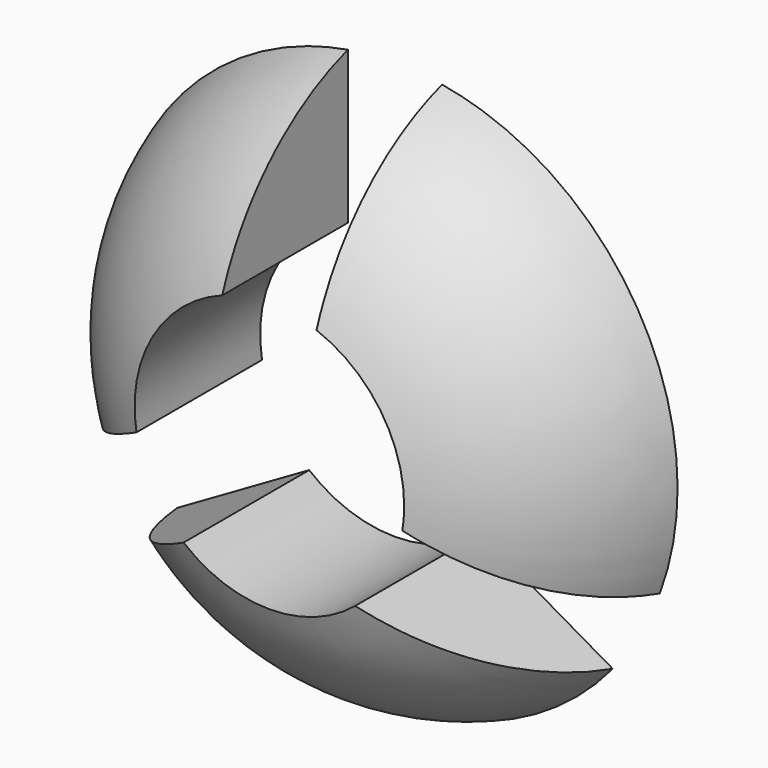
from build123d import *

# Parameters (mm, degrees)
F1_DEPTH      = 36.1303463578
F2_T2_ANGLE   = 324.8614295588
F2_2_T2_ANGLE = 324.8614295588
F2_3_T2_ANGLE = 324.8614295588
F3_T          = -2.54
F3_2_T        = -2.54
F3_3_T        = -2.54


# Not quite as in the source:
# - a fillet or chamfer that OpenCascade refuses, or shapes differently, is made with other operations: its cross-section is extruded or revolved along the edge and cut away or added


with BuildPart() as f1:
    # F0 (on Front) → F1 (new body)
    with BuildSketch(Plane.XZ):
        with BuildLine():
            Line((-10.8511227613, 29.0617289596), (-10.8511227613, 66.6497174079))
            ThreePointArc((-10.8511227613, 66.6497174079), (-58.4803280753, 33.7636331566), (-63.1459098109, -23.9275107331))
            Line((-63.1459098109, -23.9275107331), (-30.5937569375, -5.133516509))
            ThreePointArc((-30.5937569375, -5.133516509), (-26.8653720703, 15.5107297967), (-10.8511227613, 29.0617289596))
        make_face()
    extrude(amount=F1_DEPTH)

    # F2: fillet of radius 56.1783848041 on 1 edges, made by hand

    # F2_s1 → F2_t2 (revolve, cut)
    with BuildSketch(Plane(origin=(0, 0, 0), x_dir=(0, 1, 0), z_dir=(-0.2152588649, 0, -0.976557024))):
        with BuildLine():
            ThreePointArc((16.4909477227, 67.5272663131), (-15.5312106796, 57.5072208472), (-36.1303463578, 31.0214595933))
            Line((-36.1303463578, 31.0214595933), (-37.1827722394, 31.414911155))
            ThreePointArc((-37.1827722394, 31.414911155), (-37.2539140539, 49.2743629532), (-37.2539140539, 67.5272663131))
            Line((-37.2539140539, 67.5272663131), (-36.1303463578, 68.6508340092))
            Line((-36.1303463578, 68.6508340092), (16.4909477227, 68.6508340092))
            Line((16.4909477227, 68.6508340092), (16.4909477227, 67.5272663131))
        make_face()
    revolve(axis=Axis((0, -36.1303463578, 0), (0, -1, 0)), revolution_arc=F2_T2_ANGLE, mode=Mode.SUBTRACT)

    # F3
    f3_openings = [f1.faces().sort_by_distance(p)[0] for p in [
        (-38.951451, 0, 22.488629),
    ]]
    offset(amount=F3_T, openings=f3_openings, kind=Kind.INTERSECTION)


with BuildPart() as f1b:
    # F0 (on Front) → F1, piece 2 (new body)
    with BuildSketch(Plane.XZ):
        with BuildLine():
            ThreePointArc((63.1459098109, -23.9275107331), (66.4228965196, -12.1626688548), (67.5272663131, 0))
            ThreePointArc((67.5272663131, 0), (51.4425813516, 43.7446284658), (10.8511227613, 66.6497174079))
            Line((10.8511227613, 66.6497174079), (10.8511227613, 29.0617289596))
            ThreePointArc((10.8511227613, 29.0617289596), (25.484785869, 17.6877540833), (31.0214595933, 0))
            ThreePointArc((31.0214595933, 0), (30.9143490142, -2.5756514375), (30.5937569375, -5.133516509))
            Line((30.5937569375, -5.133516509), (63.1459098109, -23.9275107331))
        make_face()
    extrude(amount=F1_DEPTH)

    # F2#2: fillet of radius 56.1783848041 on 1 edges, made by hand

    # F2_2_s1 → F2_2_t2 (revolve, cut)
    with BuildSketch(Plane(origin=(0, 0, 0), x_dir=(0, 1, 0), z_dir=(0.2152588649, 0, -0.976557024))):
        with BuildLine():
            ThreePointArc((-36.1303463578, -31.0214595933), (-15.5312106796, -57.5072208472), (16.4909477227, -67.5272663131))
            Line((16.4909477227, -67.5272663131), (-36.1303463578, -67.5272663131))
            Line((-36.1303463578, -67.5272663131), (-36.1303463578, -31.0214595933))
        make_face()
    revolve(axis=Axis((0, -36.1303463578, 0), (0, 1, 0)), revolution_arc=F2_2_T2_ANGLE, mode=Mode.SUBTRACT)

    # F3#3
    f3_3_openings = [f1b.faces().sort_by_distance(p)[0] for p in [
        (38.951451, 0, 22.488652),
    ]]
    offset(amount=F3_3_T, openings=f3_3_openings, kind=Kind.INTERSECTION)


with BuildPart() as f1c:
    # F0 (on Front) → F1, piece 3 (new body)
    with BuildSketch(Plane.XZ):
        with BuildLine():
            ThreePointArc((-52.2947870496, -42.7222066748), (0, -67.5272663131), (52.2947870496, -42.7222066748))
            Line((52.2947870496, -42.7222066748), (19.7426341763, -23.9282124506))
            ThreePointArc((19.7426341763, -23.9282124506), (0, -31.0214595933), (-19.7426341763, -23.9282124506))
            Line((-19.7426341763, -23.9282124506), (-52.2947870496, -42.7222066748))
        make_face()
    extrude(amount=F1_DEPTH)

    # F2#3: fillet of radius 56.1783848041 on 1 edges, made by hand

    # F2_3_s1 → F2_3_t2 (revolve, cut)
    with BuildSketch(Plane(origin=(0, 0, 0), x_dir=(0, 1, 0), z_dir=(0.9533526235, 0, 0.3018588666))):
        with BuildLine():
            ThreePointArc((16.4909477227, 67.5272663131), (-15.5312106796, 57.5072208472), (-36.1303463578, 31.0214595933))
            Line((-36.1303463578, 31.0214595933), (-37.1827722394, 31.414911155))
            ThreePointArc((-37.1827722394, 31.414911155), (-37.2539140539, 49.2743629532), (-37.2539140539, 67.5272663131))
            Line((-37.2539140539, 67.5272663131), (-36.1303463578, 68.6508340092))
            Line((-36.1303463578, 68.6508340092), (16.4909477227, 68.6508340092))
            Line((16.4909477227, 68.6508340092), (16.4909477227, 67.5272663131))
        make_face()
    revolve(axis=Axis((0, -36.1303463578, 0), (0, -1, 0)), revolution_arc=F2_3_T2_ANGLE, mode=Mode.SUBTRACT)

    # F3#2
    f3_2_openings = [f1c.faces().sort_by_distance(p)[0] for p in [
        (-4e-06, 0, -44.977268),
    ]]
    offset(amount=F3_2_T, openings=f3_2_openings, kind=Kind.INTERSECTION)


solid = Compound([f1.part, f1b.part, f1c.part])
